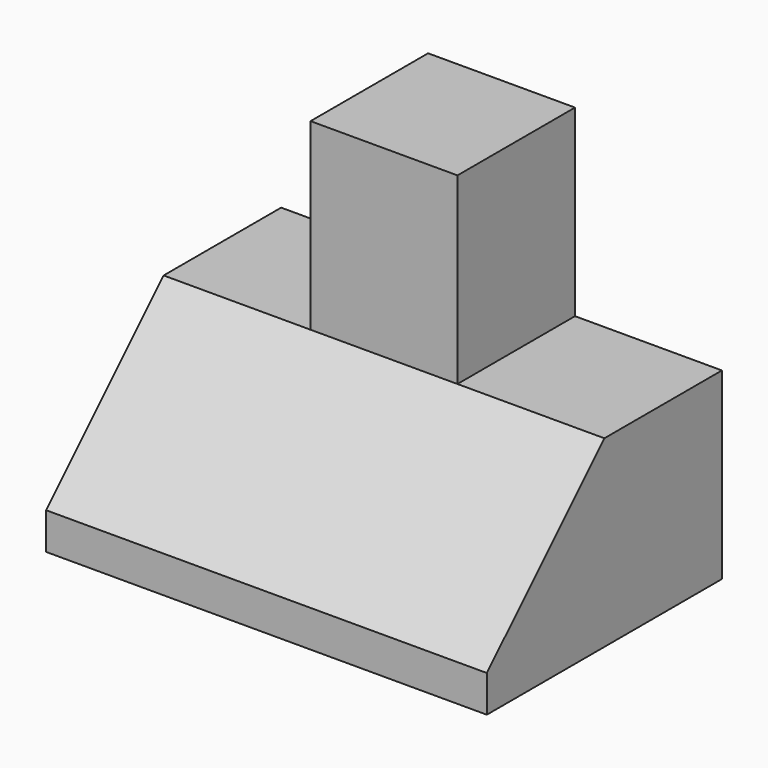
from build123d import *

# Parameters (mm, degrees)
F0_W     = 600
F0_H     = 400
F1_DEPTH = 250
F2_W     = 200
F2_H     = 200
F3_DEPTH = 250
F4_SIZE  = 199.99999


# Not quite as in the source:
# - a fillet or chamfer is up to 0.001 mm smaller than in the source, because OpenCascade refuses the exact size


with BuildPart() as f1:
    # F0 (on Top) → F1 (new body)
    with BuildSketch(Plane.XY):
        Rectangle(F0_W, F0_H)
    extrude(amount=F1_DEPTH)

    # F2 (on face) → F3 (join)
    with BuildSketch(Plane.XY.offset(250)):
        with Locations((0, 100)):
            Rectangle(F2_W, F2_H)
    extrude(amount=F3_DEPTH)

    # F4 (size 200 in the source; OpenCascade refuses exactly that, so slightly less here)
    f4_edges = [f1.edges().sort_by_distance(p)[0] for p in [
        (0, -200, 250),
    ]]
    chamfer(f4_edges, length=F4_SIZE)


solid = f1.part
